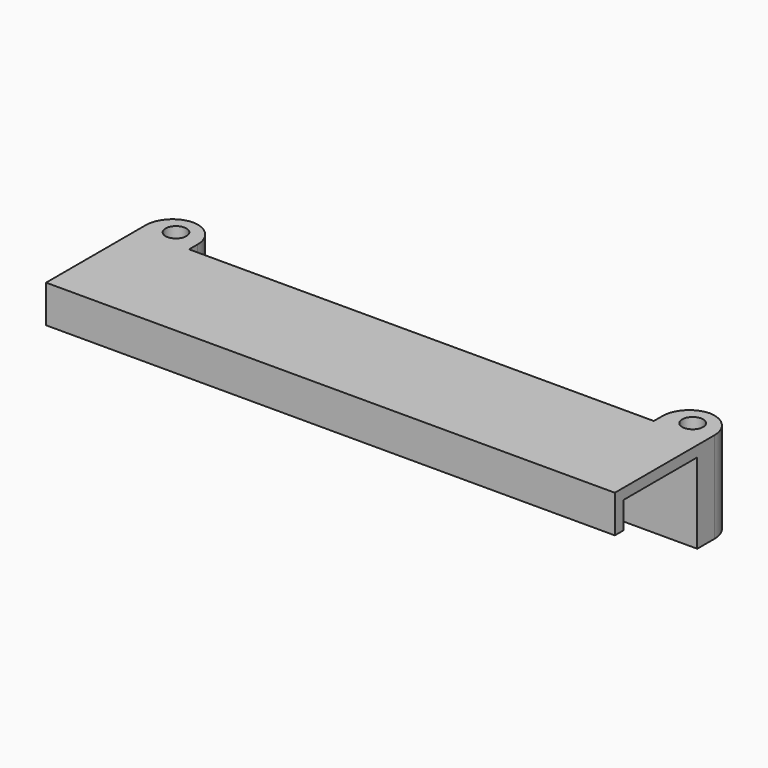
from build123d import *

# Parameters (mm, degrees)
F1_DEPTH    = 53
F2_W        = 9.7
F2_H        = 17
F3_DEPTH    = 7
F4_R        = 1.95
F5_DEPTH    = 25
F6_T1_DEPTH = 42
F7_R        = 1.95
F8_DEPTH    = 7


# Not quite as in the source:
# - a fillet or chamfer that OpenCascade refuses, or shapes differently, is made with other operations: its cross-section is extruded or revolved along the edge and cut away or added
# - a pattern or mirror of a feature is missing from the dataset's text; its kind, count and spacing are read off the source's solid


with BuildPart() as f1:
    # F0 (on Right) → F1 (new body, symmetric)
    with BuildSketch(Plane.YZ):
        Polygon((-17.2, 0), (0, 0), (0, -15), (2, -15), (2, 2), (-19.2, 2), (-19.2, -5), (-17.2, -5), align=None)
    extrude(amount=F1_DEPTH, both=True)

    # F2 (on face) → F3 (join)
    with BuildSketch(Plane(origin=(0, 2, 0), x_dir=(-1, 0, 0), z_dir=(0, 1, 0))):
        with Locations((-48.15, -6.5)):
            Rectangle(F2_W, F2_H)
    f3 = extrude(amount=F3_DEPTH)

    # F3_copies: F3 across plane
    add(f3.mirror(Plane(origin=(0, 0, 0), x_dir=(0, 0, -1), z_dir=(-1, 0, 0))))

    # F4 (on face) → F5 (cut)
    with BuildSketch(Plane.XY.offset(2)):
        with Locations((48.15, 5)):
            Circle(F4_R)
    f5 = extrude(amount=-F5_DEPTH, mode=Mode.SUBTRACT)

    # F5_copies: F5 across plane
    add(f5.mirror(Plane(origin=(0, 0, 0), x_dir=(0, 0, -1), z_dir=(-1, 0, 0))), mode=Mode.SUBTRACT)

    # F6: fillet of radius 5 on 4 edges, made by hand

    # F6_s2 → F6_t1 (cut)
    with BuildSketch(Plane.XY.offset(-27.5)):
        with BuildLine():
            ThreePointArc((53, 4), (51.5355339059, 7.5355339059), (48, 9))
            Line((48, 9), (53, 9))
            Line((53, 9), (53, 4))
        make_face()
        with BuildLine():
            ThreePointArc((48.3, 9), (44.7644660941, 7.5355339059), (43.3, 4))
            Line((43.3, 4), (43.3, 9))
            Line((43.3, 9), (48.3, 9))
        make_face()
        with BuildLine():
            ThreePointArc((-53, 4), (-51.5355339059, 7.5355339059), (-48, 9))
            Line((-48, 9), (-53, 9))
            Line((-53, 9), (-53, 4))
        make_face()
        with BuildLine():
            ThreePointArc((-48.3, 9), (-44.7644660941, 7.5355339059), (-43.3, 4))
            Line((-43.3, 4), (-43.3, 9))
            Line((-43.3, 9), (-48.3, 9))
        make_face()
    extrude(amount=F6_T1_DEPTH, mode=Mode.SUBTRACT)

    # F7 (on face) → F8 (join)
    with BuildSketch(Plane(origin=(0, 0, -15), x_dir=(1, 0, 0), z_dir=(0, 0, -1))):
        with Locations((48.15, -5)):
            Circle(F7_R)
    f8 = extrude(amount=-F8_DEPTH)

    # F8_copies: F8 across plane
    add(f8.mirror(Plane(origin=(0, 0, 0), x_dir=(0, 0, -1), z_dir=(-1, 0, 0))))


solid = f1.part
